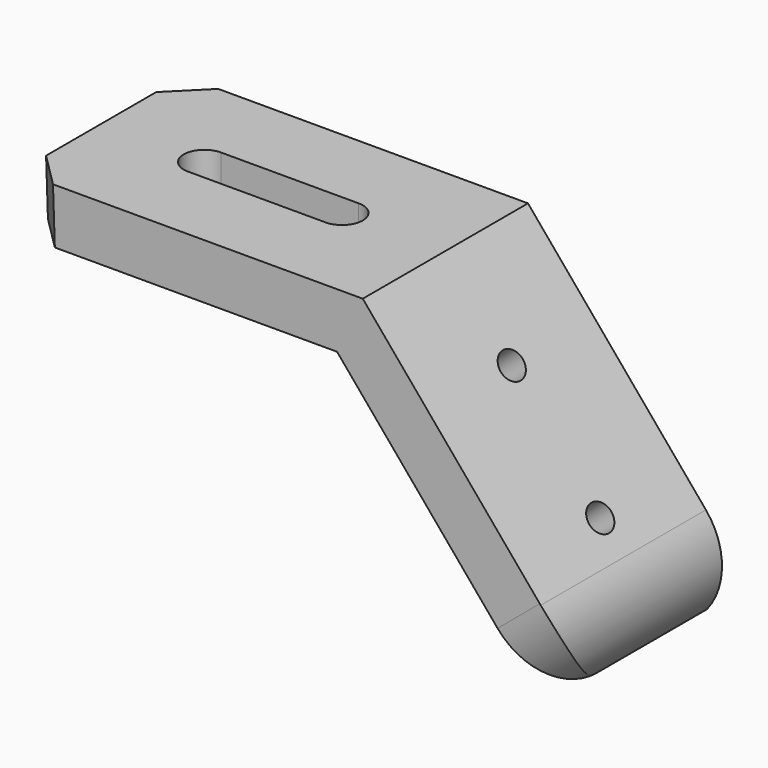
from build123d import *

# Parameters (mm, degrees)
F1_DEPTH    = 15
F3_DEPTH    = 43.4455230334
F5_D        = 4
F6_T1_DEPTH = 78.9897948557
F6_T3_DEPTH = 58
F7_SIZE     = 5


# Not quite as in the source:
# - a fillet or chamfer that OpenCascade refuses, or shapes differently, is made with other operations: its cross-section is extruded or revolved along the edge and cut away or added


with BuildPart() as f1:
    # F0 (on Front) → F1 (new body, symmetric)
    with BuildSketch(Plane.XZ):
        Polygon((-0.2695387348, 8), (0, 0), (46, 0), (75.7414862046, -35.4445230334), (81.8698417496, -30.3022221559), (49.7304612652, 8), align=None)
    extrude(amount=F1_DEPTH, both=True)

    # F2 (on face) → F3 (cut, through all)
    with BuildSketch(Plane.XY.offset(8)):
        with BuildLine():
            ThreePointArc((14.7304612652, 3), (11.7304612652, 0), (14.7304612652, -3))
            Line((14.7304612652, -3), (34.7304612652, -3))
            ThreePointArc((34.7304612652, -3), (37.7304612652, 0), (34.7304612652, 3))
            Line((34.7304612652, 3), (14.7304612652, 3))
        make_face()
    extrude(amount=-F3_DEPTH, mode=Mode.SUBTRACT)

    # F5 (through all)
    with Locations(Plane(origin=(33.1222636313, 0, 27.7928791968), x_dir=(0, 1, 0), z_dir=(0.7660444431, 0, 0.6427876097))):
        with Locations((0, -40.8377687803), (0, -60.8377687803)):
            Hole(F5_D / 2)

    # F6: fillet of radius 10 on 2 edges, made by hand

    # F6_s2 → F6_t1 (cut)
    with BuildSketch(Plane.XZ.offset(-39.4948974278)):
        with BuildLine():
            ThreePointArc((75.7414862046, -35.4445230334), (77.9104912295, -29.0903052725), (75.5718351227, -22.7965501322))
            Line((75.5718351227, -22.7965501322), (81.8698417496, -30.3022221559))
            Line((81.8698417496, -30.3022221559), (75.7414862046, -35.4445230334))
        make_face()
    extrude(amount=F6_T1_DEPTH, mode=Mode.SUBTRACT)

    # F6_s4 → F6_t3 (cut)
    with BuildSketch(Plane(origin=(7.8427970084, 0, 6.5808880771), x_dir=(0, 1, 0), z_dir=(0.7660444431, 0, 0.6427876097))):
        with BuildLine():
            ThreePointArc((-15, -65.8377687803), (-12.0710678119, -72.9088365922), (-5, -75.8377687803))
            Line((-5, -75.8377687803), (-15, -75.8377687803))
            Line((-15, -75.8377687803), (-15, -65.8377687803))
        make_face()
    extrude(amount=F6_T3_DEPTH, mode=Mode.SUBTRACT)

    # F7
    f7_edges = [f1.edges().sort_by_distance(p)[0] for p in [
        (-0.134769, -15, 4),
        (-0.134769, 15, 4),
    ]]
    chamfer(f7_edges, length=F7_SIZE)


solid = f1.part
